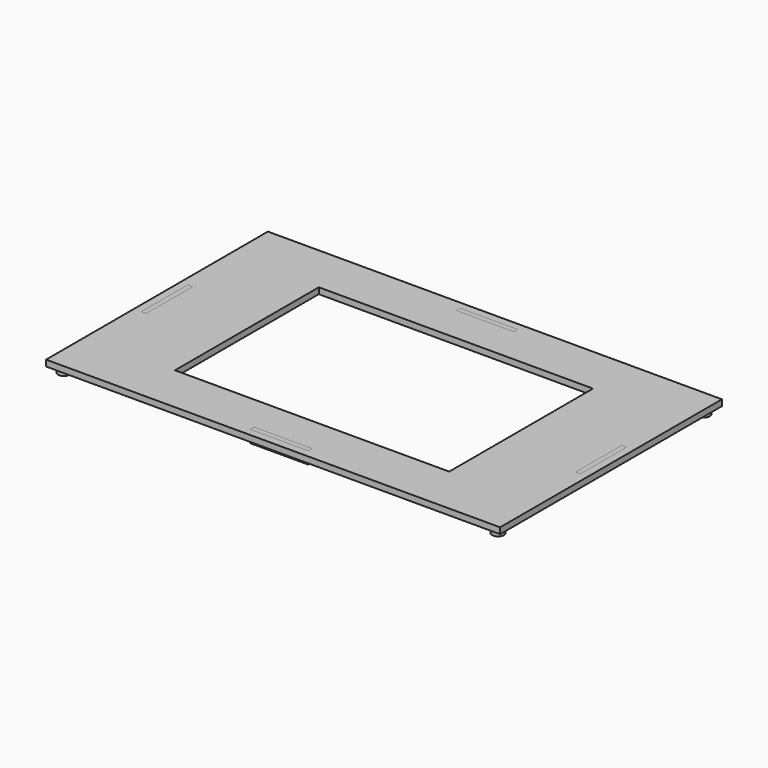
from build123d import *

# Parameters (mm, degrees)
F1_DEPTH = 2
F2_DEPTH = 5
F3_DEPTH = 2
F0_W     = 1.6
F0_H     = 9.5
F0_W_2   = 9.5
F0_H_2   = 1.6
F4_DEPTH = 2


# Not quite as in the source:
# - a feature names something its author has since deleted; it is built from what else it names


with BuildPart() as f1:
    # F0 (on Top) → F1 (new body)
    with BuildSketch(Plane.XY):
        with BuildLine():
            Line((72.6288582233, -43.6288582233), (74.5, -45.5))
            Line((74.5, -45.5), (74.5, 0))
            Line((74.5, 0), (72.05, 0))
            Line((72.05, 0), (72.05, -9.5))
            Line((72.05, -9.5), (70.45, -9.5))
            Line((70.45, -9.5), (70.45, 0))
            Line((70.45, 0), (68, 0))
            Line((68, 0), (68, -39))
            Line((68, -39), (69.8711417767, -40.8711417767))
            ThreePointArc((69.8711417767, -40.8711417767), (71.9962326931, -40.4484349116), (73.2, -42.25))
            ThreePointArc((73.2, -42.25), (73.0515650884, -42.9962326931), (72.6288582233, -43.6288582233))
        make_face()
        with BuildLine():
            Line((0, -45.5), (74.5, -45.5))
            Line((74.5, -45.5), (72.6288582233, -43.6288582233))
            ThreePointArc((72.6288582233, -43.6288582233), (69.8711417767, -43.6288582233), (69.8711417767, -40.8711417767))
            Line((69.8711417767, -40.8711417767), (68, -39))
            Line((68, -39), (0, -39))
            Line((0, -39), (0, -41.45))
            Line((0, -41.45), (9.5, -41.45))
            Line((9.5, -41.45), (9.5, -43.05))
            Line((9.5, -43.05), (0, -43.05))
            Line((0, -43.05), (0, -45.5))
        make_face()
        with BuildLine():
            Line((-74.5, -45.5), (0, -45.5))
            Line((0, -45.5), (0, -43.05))
            Line((0, -43.05), (-9.5, -43.05))
            Line((-9.5, -43.05), (-9.5, -41.45))
            Line((-9.5, -41.45), (0, -41.45))
            Line((0, -41.45), (0, -39))
            Line((0, -39), (-68, -39))
            Line((-68, -39), (-69.8711417767, -40.8711417767))
            ThreePointArc((-69.8711417767, -40.8711417767), (-69.4484349116, -41.5037673069), (-69.3, -42.25))
            ThreePointArc((-69.3, -42.25), (-70.5037673069, -44.0515650884), (-72.6288582233, -43.6288582233))
            Line((-72.6288582233, -43.6288582233), (-74.5, -45.5))
        make_face()
        with BuildLine():
            Line((72.05, 0), (74.5, 0))
            Line((74.5, 0), (74.5, 45.5))
            Line((74.5, 45.5), (72.6288582233, 43.6288582233))
            ThreePointArc((72.6288582233, 43.6288582233), (73.0515650884, 42.9962326931), (73.2, 42.25))
            ThreePointArc((73.2, 42.25), (71.9962326931, 40.4484349116), (69.8711417767, 40.8711417767))
            Line((69.8711417767, 40.8711417767), (68, 39))
            Line((68, 39), (68, 0))
            Line((68, 0), (70.45, 0))
            Line((70.45, 0), (70.45, 9.5))
            Line((70.45, 9.5), (72.05, 9.5))
            Line((72.05, 9.5), (72.05, 0))
        make_face()
        with BuildLine():
            ThreePointArc((69.8711417767, -40.8711417767), (69.8711417767, -43.6288582233), (72.6288582233, -43.6288582233))
            Line((72.6288582233, -43.6288582233), (69.8711417767, -40.8711417767))
        make_face()
        with BuildLine():
            Line((69.8711417767, -40.8711417767), (72.6288582233, -43.6288582233))
            ThreePointArc((72.6288582233, -43.6288582233), (73.0515650884, -42.9962326931), (73.2, -42.25))
            ThreePointArc((73.2, -42.25), (71.9962326931, -40.4484349116), (69.8711417767, -40.8711417767))
        make_face()
        with BuildLine():
            Line((-74.5, 0), (-74.5, -45.5))
            Line((-74.5, -45.5), (-72.6288582233, -43.6288582233))
            ThreePointArc((-72.6288582233, -43.6288582233), (-72.6288582233, -40.8711417767), (-69.8711417767, -40.8711417767))
            Line((-69.8711417767, -40.8711417767), (-68, -39))
            Line((-68, -39), (-68, 0))
            Line((-68, 0), (-70.45, 0))
            Line((-70.45, 0), (-70.45, -9.5))
            Line((-70.45, -9.5), (-72.05, -9.5))
            Line((-72.05, -9.5), (-72.05, 0))
            Line((-72.05, 0), (-74.5, 0))
        make_face()
        with BuildLine():
            Line((72.6288582233, 43.6288582233), (74.5, 45.5))
            Line((74.5, 45.5), (0, 45.5))
            Line((0, 45.5), (0, 43.05))
            Line((0, 43.05), (9.5, 43.05))
            Line((9.5, 43.05), (9.5, 41.45))
            Line((9.5, 41.45), (0, 41.45))
            Line((0, 41.45), (0, 39))
            Line((0, 39), (68, 39))
            Line((68, 39), (69.8711417767, 40.8711417767))
            ThreePointArc((69.8711417767, 40.8711417767), (69.8711417767, 43.6288582233), (72.6288582233, 43.6288582233))
        make_face()
        with BuildLine():
            Line((-74.5, 45.5), (-74.5, 0))
            Line((-74.5, 0), (-72.05, 0))
            Line((-72.05, 0), (-72.05, 9.5))
            Line((-72.05, 9.5), (-70.45, 9.5))
            Line((-70.45, 9.5), (-70.45, 0))
            Line((-70.45, 0), (-68, 0))
            Line((-68, 0), (-68, 39))
            Line((-68, 39), (-69.8711417767, 40.8711417767))
            ThreePointArc((-69.8711417767, 40.8711417767), (-72.6288582233, 40.8711417767), (-72.6288582233, 43.6288582233))
            Line((-72.6288582233, 43.6288582233), (-74.5, 45.5))
        make_face()
        with BuildLine():
            ThreePointArc((-69.8711417767, -40.8711417767), (-72.6288582233, -40.8711417767), (-72.6288582233, -43.6288582233))
            Line((-72.6288582233, -43.6288582233), (-69.8711417767, -40.8711417767))
        make_face()
        with BuildLine():
            Line((-69.8711417767, -40.8711417767), (-72.6288582233, -43.6288582233))
            ThreePointArc((-72.6288582233, -43.6288582233), (-70.5037673069, -44.0515650884), (-69.3, -42.25))
            ThreePointArc((-69.3, -42.25), (-69.4484349116, -41.5037673069), (-69.8711417767, -40.8711417767))
        make_face()
        with BuildLine():
            Line((0, 43.05), (0, 45.5))
            Line((0, 45.5), (-74.5, 45.5))
            Line((-74.5, 45.5), (-72.6288582233, 43.6288582233))
            ThreePointArc((-72.6288582233, 43.6288582233), (-70.5037673069, 44.0515650884), (-69.3, 42.25))
            ThreePointArc((-69.3, 42.25), (-69.4484349116, 41.5037673069), (-69.8711417767, 40.8711417767))
            Line((-69.8711417767, 40.8711417767), (-68, 39))
            Line((-68, 39), (0, 39))
            Line((0, 39), (0, 41.45))
            Line((0, 41.45), (-9.5, 41.45))
            Line((-9.5, 41.45), (-9.5, 43.05))
            Line((-9.5, 43.05), (0, 43.05))
        make_face()
        with BuildLine():
            ThreePointArc((73.2, 42.25), (73.0515650884, 42.9962326931), (72.6288582233, 43.6288582233))
            Line((72.6288582233, 43.6288582233), (69.8711417767, 40.8711417767))
            ThreePointArc((69.8711417767, 40.8711417767), (71.9962326931, 40.4484349116), (73.2, 42.25))
        make_face()
        with BuildLine():
            Line((69.8711417767, 40.8711417767), (72.6288582233, 43.6288582233))
            ThreePointArc((72.6288582233, 43.6288582233), (69.8711417767, 43.6288582233), (69.8711417767, 40.8711417767))
        make_face()
        Polygon((0, -39), (68, -39), (68, 0), (45, 0), (45, -29.5), (0, -29.5), align=None)
        Polygon((-68, -39), (0, -39), (0, -29.5), (-45, -29.5), (-45, 0), (-68, 0), align=None)
        Polygon((45, 0), (68, 0), (68, 39), (0, 39), (0, 29.5), (45, 29.5), align=None)
        with BuildLine():
            ThreePointArc((-69.3, 42.25), (-70.5037673069, 44.0515650884), (-72.6288582233, 43.6288582233))
            Line((-72.6288582233, 43.6288582233), (-69.8711417767, 40.8711417767))
            ThreePointArc((-69.8711417767, 40.8711417767), (-69.4484349116, 41.5037673069), (-69.3, 42.25))
        make_face()
        with BuildLine():
            Line((-69.8711417767, 40.8711417767), (-72.6288582233, 43.6288582233))
            ThreePointArc((-72.6288582233, 43.6288582233), (-72.6288582233, 40.8711417767), (-69.8711417767, 40.8711417767))
        make_face()
        Polygon((-45, -29.5), (0, -29.5), (45, -29.5), (45, 0), (45, 29.5), (0, 29.5), (-45, 29.5), (-45, 0), align=None)
        Polygon((-68, 39), (-68, 0), (-45, 0), (-45, 29.5), (0, 29.5), (0, 39), align=None)
    extrude(amount=F1_DEPTH)

    # F0 (on Top) → F2 (cut)
    with BuildSketch(Plane.XY):
        Polygon((-45, -29.5), (0, -29.5), (45, -29.5), (45, 0), (45, 29.5), (0, 29.5), (-45, 29.5), (-45, 0), align=None)
    extrude(amount=F2_DEPTH, mode=Mode.SUBTRACT)

    # F0 (on Top) → F3 (join)
    with BuildSketch(Plane.XY):
        with BuildLine():
            ThreePointArc((73.2, 42.25), (73.0515650884, 42.9962326931), (72.6288582233, 43.6288582233))
            Line((72.6288582233, 43.6288582233), (69.8711417767, 40.8711417767))
            ThreePointArc((69.8711417767, 40.8711417767), (71.9962326931, 40.4484349116), (73.2, 42.25))
        make_face()
        with BuildLine():
            Line((69.8711417767, 40.8711417767), (72.6288582233, 43.6288582233))
            ThreePointArc((72.6288582233, 43.6288582233), (69.8711417767, 43.6288582233), (69.8711417767, 40.8711417767))
        make_face()
        with BuildLine():
            Line((-69.8711417767, 40.8711417767), (-72.6288582233, 43.6288582233))
            ThreePointArc((-72.6288582233, 43.6288582233), (-72.6288582233, 40.8711417767), (-69.8711417767, 40.8711417767))
        make_face()
        with BuildLine():
            ThreePointArc((-69.3, 42.25), (-70.5037673069, 44.0515650884), (-72.6288582233, 43.6288582233))
            Line((-72.6288582233, 43.6288582233), (-69.8711417767, 40.8711417767))
            ThreePointArc((-69.8711417767, 40.8711417767), (-69.4484349116, 41.5037673069), (-69.3, 42.25))
        make_face()
        with BuildLine():
            Line((-69.8711417767, -40.8711417767), (-72.6288582233, -43.6288582233))
            ThreePointArc((-72.6288582233, -43.6288582233), (-70.5037673069, -44.0515650884), (-69.3, -42.25))
            ThreePointArc((-69.3, -42.25), (-69.4484349116, -41.5037673069), (-69.8711417767, -40.8711417767))
        make_face()
        with BuildLine():
            ThreePointArc((-69.8711417767, -40.8711417767), (-72.6288582233, -40.8711417767), (-72.6288582233, -43.6288582233))
            Line((-72.6288582233, -43.6288582233), (-69.8711417767, -40.8711417767))
        make_face()
        with BuildLine():
            ThreePointArc((69.8711417767, -40.8711417767), (69.8711417767, -43.6288582233), (72.6288582233, -43.6288582233))
            Line((72.6288582233, -43.6288582233), (69.8711417767, -40.8711417767))
        make_face()
        with BuildLine():
            Line((69.8711417767, -40.8711417767), (72.6288582233, -43.6288582233))
            ThreePointArc((72.6288582233, -43.6288582233), (73.0515650884, -42.9962326931), (73.2, -42.25))
            ThreePointArc((73.2, -42.25), (71.9962326931, -40.4484349116), (69.8711417767, -40.8711417767))
        make_face()
    extrude(amount=-F3_DEPTH)


with BuildPart() as f3:
    # F0 (on Top) → F3, piece 2 (new body)
    with BuildSketch(Plane.XY):
        with Locations((-71.25, -4.75)):
            Rectangle(F0_W, F0_H)
        with Locations((-71.25, 4.75)):
            Rectangle(F0_W, F0_H)
    extrude(amount=-F3_DEPTH)


with BuildPart() as f3b:
    # F0 (on Top) → F3, piece 3 (new body)
    with BuildSketch(Plane.XY):
        with Locations((-4.75, 42.25)):
            Rectangle(F0_W_2, F0_H_2)
        with Locations((4.75, 42.25)):
            Rectangle(F0_W_2, F0_H_2)
    extrude(amount=-F3_DEPTH)


with BuildPart() as f3c:
    # F0 (on Top) → F3, piece 4 (new body)
    with BuildSketch(Plane.XY):
        with Locations((71.25, 4.75)):
            Rectangle(F0_W, F0_H)
        with Locations((71.25, -4.75)):
            Rectangle(F0_W, F0_H)
    extrude(amount=-F3_DEPTH)


with BuildPart() as f3d:
    # F0 (on Top) → F3, piece 5 (new body)
    with BuildSketch(Plane.XY):
        with Locations((4.75, -42.25)):
            Rectangle(F0_W_2, F0_H_2)
        with Locations((-4.75, -42.25)):
            Rectangle(F0_W_2, F0_H_2)
    extrude(amount=-F3_DEPTH)


with BuildPart() as f4:
    # F0 (on Top) → F4 (new body)
    with BuildSketch(Plane.XY):
        with Locations((-4.75, 42.25)):
            Rectangle(F0_W_2, F0_H_2)
        with Locations((4.75, 42.25)):
            Rectangle(F0_W_2, F0_H_2)
    extrude(amount=F4_DEPTH)


with BuildPart() as f4b:
    # F0 (on Top) → F4, piece 2 (new body)
    with BuildSketch(Plane.XY):
        with Locations((-71.25, 4.75)):
            Rectangle(F0_W, F0_H)
        with Locations((-71.25, -4.75)):
            Rectangle(F0_W, F0_H)
    extrude(amount=F4_DEPTH)


with BuildPart() as f4c:
    # F0 (on Top) → F4, piece 3 (new body)
    with BuildSketch(Plane.XY):
        with Locations((71.25, 4.75)):
            Rectangle(F0_W, F0_H)
        with Locations((71.25, -4.75)):
            Rectangle(F0_W, F0_H)
    extrude(amount=F4_DEPTH)


with BuildPart() as f4d:
    # F0 (on Top) → F4, piece 4 (new body)
    with BuildSketch(Plane.XY):
        with Locations((-4.75, -42.25)):
            Rectangle(F0_W_2, F0_H_2)
        with Locations((4.75, -42.25)):
            Rectangle(F0_W_2, F0_H_2)
    extrude(amount=F4_DEPTH)


solid = Compound([f1.part, f3.part, f3b.part, f3c.part, f3d.part, f4.part, f4b.part, f4c.part, f4d.part])
